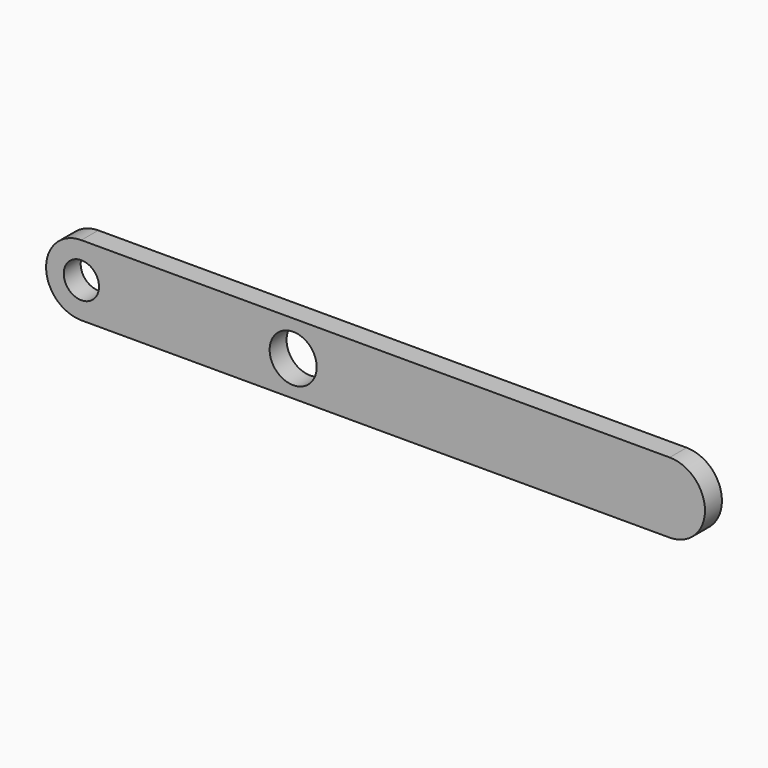
from build123d import *

# Parameters (mm, degrees)
F1_DEPTH = 3.6
F2_R     = 3
F3_DEPTH = 3.6
F4_R     = 4
F5_DEPTH = 3.601


# Not quite as in the source:
# - a feature names something its author has since deleted; it is built from what else it names


with BuildPart() as f1:
    # F0 (on Front) → F1 (new body)
    with BuildSketch(Plane.XZ):
        with BuildLine():
            Line((50, 6), (-50, 6))
            ThreePointArc((-50, 6), (-56, 0), (-50, -6))
            Line((-50, -6), (50, -6))
            ThreePointArc((50, -6), (56, 0), (50, 6))
        make_face()
    extrude(amount=F1_DEPTH)

    # F2 (on face) → F3 (cut, through all)
    with BuildSketch(Plane.XZ.offset(3.6)):
        with Locations((-50, 0)):
            Circle(F2_R)
    extrude(amount=-F3_DEPTH, mode=Mode.SUBTRACT)

    # F4 (on face) → F5 (cut, through all)
    with BuildSketch(Plane.XZ.offset(3.6)):
        with Locations((-14, 0)):
            Circle(F4_R)
    extrude(amount=-F5_DEPTH, mode=Mode.SUBTRACT)


solid = f1.part
